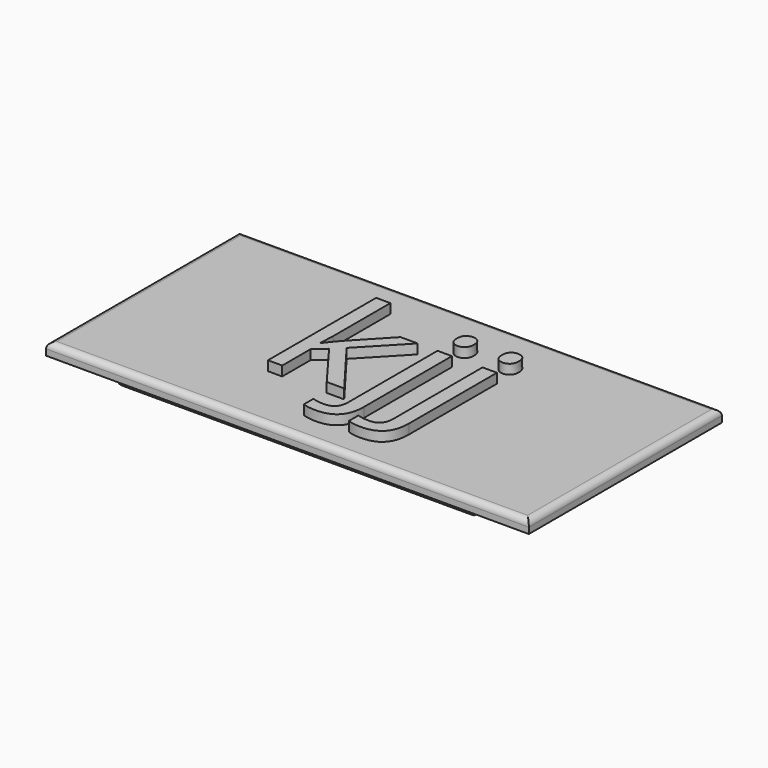
from build123d import *

# Parameters (mm, degrees)
F0_W         = 400
F0_H         = 200
F1_DEPTH     = 10
F2_W         = 300
F2_H         = 180
F3_DEPTH     = 8
F4_R         = 5
F5_R         = 5
F6_TEXT_SIZE = 147.4201474201
F7_DEPTH     = 8
F8_R         = 15
F9_DEPTH     = 10


# Not quite as in the source:
# - Text() gives the source's letters only with a copy of the font that has no kerning and outlines rounded to 1/6400 em; it was checked with that copy


with BuildPart() as f1:
    # F0 (on Top) → F1 (new body)
    with BuildSketch(Plane.XY):
        Rectangle(F0_W, F0_H)
    extrude(amount=F1_DEPTH)

    # F2 (on Top) → F3 (join)
    with BuildSketch(Plane.XY):
        Rectangle(F2_W, F2_H)
    extrude(amount=-F3_DEPTH)

    # F4
    f4_edges = [f1.edges().sort_by_distance(p)[0] for p in [
        (0, 100, 10),
        (-200, 0, 10),
        (0, -100, 10),
        (200, 0, 10),
    ]]
    fillet(f4_edges, radius=F4_R)

    # F5
    f5_edges = [f1.edges().sort_by_distance(p)[0] for p in [
        (-150, 0, -8),
        (0, 90, -8),
        (150, 0, -8),
    ]]
    fillet(f5_edges, radius=F5_R)

    # F6 (on face) → F7 (join)
    with BuildSketch(Plane.XY.offset(10)):
        with Locations((-75, -42.2604369136)):
            Text('kjj', F6_TEXT_SIZE, font='Open Sans', text_align=(TextAlign.LEFT, TextAlign.BOTTOM))
    extrude(amount=F7_DEPTH)

    # F8 (on face) → F9 (cut)
    with BuildSketch(Plane(origin=(0, 0, -8), x_dir=(1, 0, 0), z_dir=(0, 0, -1))):
        Circle(F8_R)
    extrude(amount=-F9_DEPTH, mode=Mode.SUBTRACT)


solid = f1.part
